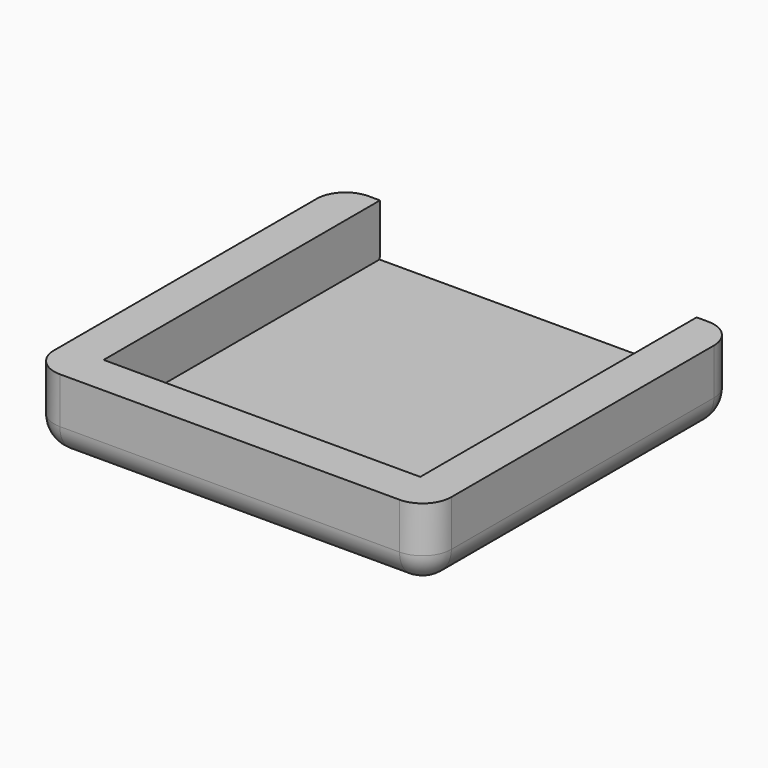
from build123d import *

# Parameters (mm, degrees)
F1_DEPTH     = 9
F0_W         = 55
F0_H         = 60
F2_DEPTH     = 4
F3_T1_DEPTH  = 74.5
F3_T3_DEPTH  = 19.5
F3_T5_DEPTH  = 92
F3_T7_DEPTH  = 91.9996386864
F3_T9_DEPTH  = 93.9999999907
F4_T1_DEPTH  = 20.5
F4_T3_DEPTH  = 20.4993548139
F4_T8_DEPTH  = 5
F4_S13_W     = 5
F4_S13_H     = 5
F4_T14_DEPTH = 5
F4_S19_W     = 5
F4_S19_H     = 5
F4_T20_DEPTH = 5
F4_S25_W     = 5
F4_S25_H     = 5
F4_T26_DEPTH = 5


# Not quite as in the source:
# - a fillet or chamfer that OpenCascade refuses, or shapes differently, is made with other operations: its cross-section is extruded or revolved along the edge and cut away or added


with BuildPart() as f1:
    # F0 (on Top) → F1 (new body)
    with BuildSketch(Plane.XY):
        Polygon((27.5, 30), (27.5, -30), (-27.5, -30), (-27.5, 30), (-34.4999999907, 29.9996386864), (-34.4999999907, -37), (34.5, -37), (34.5, 30), align=None)
    extrude(amount=F1_DEPTH)

    # F0 (on Top) → F2 (join)
    with BuildSketch(Plane.XY):
        Polygon((27.5, 30), (27.5, -30), (-27.5, -30), (-27.5, 30), (-34.4999999907, 29.9996386864), (-34.4999999907, -37), (34.5, -37), (34.5, 30), align=None)
        Rectangle(F0_W, F0_H)
    extrude(amount=-F2_DEPTH)

    # F3: fillet of radius 5 on 5 edges, made by hand

    # F3_s2 → F3_t1 (cut)
    with BuildSketch(Plane.YZ.offset(-27.5)):
        with BuildLine():
            ThreePointArc((25, -4), (28.5355339059, -2.5355339059), (30, 1))
            Line((30, 1), (30, -4))
            Line((30, -4), (25, -4))
        make_face()
    extrude(amount=F3_T1_DEPTH, mode=Mode.SUBTRACT)

    # F3_s4 → F3_t3 (cut)
    with BuildSketch(Plane(origin=(-27.4984514401, -0.0014193662, 0), x_dir=(0, 0, 1), z_dir=(-0.9999999987, -5.16162e-05, 0))):
        with BuildLine():
            ThreePointArc((-4, 25.0014194062), (-2.5355339059, 28.5369533121), (1, 30.0014194062))
            Line((1, 30.0014194062), (-4, 30.0014194062))
            Line((-4, 30.0014194062), (-4, 25.0014194062))
        make_face()
    extrude(amount=F3_T3_DEPTH, mode=Mode.SUBTRACT)

    # F3_s6 → F3_t5 (cut)
    with BuildSketch(Plane.XZ.offset(-42.5)):
        with BuildLine():
            ThreePointArc((29.5, -4), (33.0355339059, -2.5355339059), (34.5, 1))
            Line((34.5, 1), (34.5, -4))
            Line((34.5, -4), (29.5, -4))
        make_face()
    extrude(amount=F3_T5_DEPTH, mode=Mode.SUBTRACT)

    # F3_s8 → F3_t7 (cut)
    with BuildSketch(Plane.XZ.offset(-42.4996386864)):
        with BuildLine():
            ThreePointArc((-34.4999999907, 1), (-33.0355338966, -2.5355339059), (-29.4999999907, -4))
            Line((-29.4999999907, -4), (-34.4999999907, -4))
            Line((-34.4999999907, -4), (-34.4999999907, 1))
        make_face()
    extrude(amount=F3_T7_DEPTH, mode=Mode.SUBTRACT)

    # F3_s10 → F3_t9 (cut)
    with BuildSketch(Plane.YZ.offset(-46.9999999907)):
        with BuildLine():
            ThreePointArc((-32, -4), (-35.5355339059, -2.5355339059), (-37, 1))
            Line((-37, 1), (-37, -4))
            Line((-37, -4), (-32, -4))
        make_face()
    extrude(amount=F3_T9_DEPTH, mode=Mode.SUBTRACT)

    # F4: fillet of radius 5 on 4 edges, made by hand

    # F4_s2 → F4_t1 (cut)
    with BuildSketch(Plane.XY.offset(1)):
        with BuildLine():
            ThreePointArc((-34.4999999907, -32), (-33.0355338966, -35.5355339059), (-29.4999999907, -37))
            Line((-29.4999999907, -37), (-34.4999999907, -37))
            Line((-34.4999999907, -37), (-34.4999999907, -32))
        make_face()
        with BuildLine():
            ThreePointArc((29.5, -37), (33.0355339059, -35.5355339059), (34.5, -32))
            Line((34.5, -32), (34.5, -37))
            Line((34.5, -37), (29.5, -37))
        make_face()
        with BuildLine():
            ThreePointArc((34.5, 25), (33.0355339059, 28.5355339059), (29.5, 30))
            Line((29.5, 30), (34.5, 30))
            Line((34.5, 30), (34.5, 25))
        make_face()
    extrude(amount=F4_T1_DEPTH, mode=Mode.SUBTRACT)

    # F4_s4 → F4_t3 (cut)
    with BuildSketch(Plane.XY.offset(1)):
        with BuildLine():
            ThreePointArc((-34.4999999907, 24.9998967609), (-33.0356251409, 28.5353394202), (-29.5002580718, 29.9998967542))
            Line((-29.5002580718, 29.9998967542), (-34.4999999907, 29.9996386864))
            Line((-34.4999999907, 29.9996386864), (-34.4999999907, 24.9998967609))
        make_face()
    extrude(amount=F4_T3_DEPTH, mode=Mode.SUBTRACT)


with BuildPart() as f4_tool6:
    # F4_s7 → F4_t8 (new body)
    with BuildSketch(Plane.XY.offset(1)):
        Polygon((-29.4999999907, 24.9998967609), (-34.4999999907, 24.9998967609), (-34.4999999907, 29.9996386864), (-29.5002580718, 29.9998967542), align=None)
    extrude(amount=-F4_T8_DEPTH)

    # F4_s9 → F4_t10 (revolve, cut)
    with BuildSketch(Plane(origin=(-29.4999999907, 24.9998967609, 1), x_dir=(0.70712503, -0.7070885319, 0), z_dir=(0.7070885319, 0.70712503, 0))):
        with BuildLine():
            ThreePointArc((0, -5), (5, 0), (0, 5))
            Line((0, 5), (0, -5))
        make_face()
    revolve(axis=Axis((-29.4999999907, 24.9998967609, 1), (0, 0, -1)), mode=Mode.SUBTRACT)


with BuildPart() as f1_1:
    add(f1.part)

    # F4_t5: cut F4_tool6
    add(f4_tool6.part, mode=Mode.SUBTRACT)


with BuildPart() as f4_tool12:
    # F4_s13 → F4_t14 (new body)
    with BuildSketch(Plane.YZ.offset(29.5)):
        with Locations((27.5, -1.5)):
            Rectangle(F4_S13_W, F4_S13_H)
    extrude(amount=F4_T14_DEPTH)

    # F4_s15 → F4_t16 (revolve, cut)
    with BuildSketch(Plane(origin=(29.5, 25, 1), x_dir=(0, -0.7071067812, 0.7071067812), z_dir=(0, 0.7071067812, 0.7071067812))):
        with BuildLine():
            ThreePointArc((0, -5), (5, 0), (0, 5))
            Line((0, 5), (0, -5))
        make_face()
    revolve(axis=Axis((29.5, 25, 1), (1, 0, 0)), mode=Mode.SUBTRACT)


with BuildPart() as f1_2:
    add(f1_1.part)

    # F4_t11: cut F4_tool12
    add(f4_tool12.part, mode=Mode.SUBTRACT)


with BuildPart() as f4_tool18:
    # F4_s19 → F4_t20 (new body)
    with BuildSketch(Plane.XZ.offset(32)):
        with Locations((32, -1.5)):
            Rectangle(F4_S19_W, F4_S19_H)
    extrude(amount=F4_T20_DEPTH)

    # F4_s21 → F4_t22 (revolve, cut)
    with BuildSketch(Plane(origin=(29.5, -32, 1), x_dir=(-0.7071067812, 0, 0.7071067812), z_dir=(0.7071067812, 0, 0.7071067812))):
        with BuildLine():
            ThreePointArc((0, -5), (5, 0), (0, 5))
            Line((0, 5), (0, -5))
        make_face()
    revolve(axis=Axis((29.5, -32, 1), (0, -1, 0)), mode=Mode.SUBTRACT)


with BuildPart() as f1_3:
    add(f1_2.part)

    # F4_t17: cut F4_tool18
    add(f4_tool18.part, mode=Mode.SUBTRACT)


with BuildPart() as f4_tool24:
    # F4_s25 → F4_t26 (new body)
    with BuildSketch(Plane.YZ.offset(-29.4999999907)):
        with Locations((-34.5, -1.5)):
            Rectangle(F4_S25_W, F4_S25_H)
    extrude(amount=-F4_T26_DEPTH)

    # F4_s27 → F4_t28 (revolve, cut)
    with BuildSketch(Plane(origin=(-29.4999999907, -32, 1), x_dir=(0, 0.7071067812, 0.7071067812), z_dir=(0, -0.7071067812, 0.7071067812))):
        with BuildLine():
            ThreePointArc((0, -5), (5, 0), (0, 5))
            Line((0, 5), (0, -5))
        make_face()
    revolve(axis=Axis((-29.4999999907, -32, 1), (-1, 0, 0)), mode=Mode.SUBTRACT)


with BuildPart() as f1_4:
    add(f1_3.part)

    # F4_t23: cut F4_tool24
    add(f4_tool24.part, mode=Mode.SUBTRACT)


solid = f1_4.part
